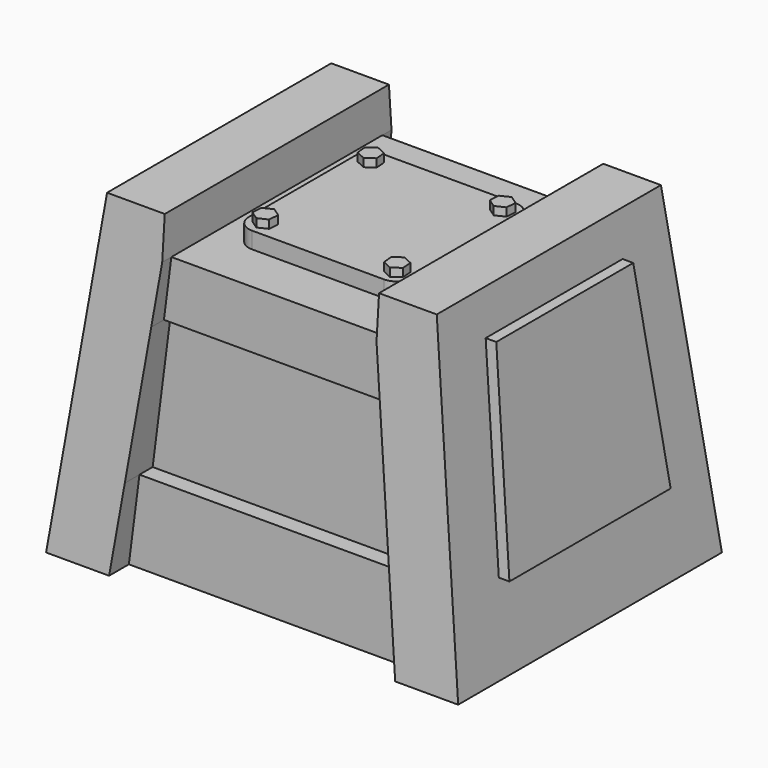
from build123d import *

# Parameters (mm, degrees)
F1_DEPTH  = 40
F2_DEPTH  = 4
F3_DEPTH  = 3
F4_DEPTH  = 5
F6_DEPTH  = 4
F7_DEPTH  = 3
F8_DEPTH  = 5
F10_DEPTH = 2
F13_DEPTH = 50
F15_DEPTH = 1
F16_DEPTH = 50
F17_DEPTH = 40


# Not quite as in the source:
# - ends of sketch curves that miss each other by under 0.0002 mm in the source are joined


with BuildPart() as f1:
    # F0 (on Front) → F1 (new body)
    with BuildSketch(Plane.XZ):
        Polygon((-20, 38.838), (-25, 0), (-17.3563005304, 0), (-16.0689015912, 10), (-13.9011792574, 26.838), (-13, 33.838), (-13, 38.838), align=None)
        Polygon((-16.0689015912, 10), (-17.3563005304, 0), (17.3563005304, 0), (16.0689015912, 10), (0, 10), align=None)
        Polygon((-13.9011792574, 26.838), (-16.0689015912, 10), (0, 10), (16.0689015912, 10), (13.9011792574, 26.838), (-3.37943e-05, 26.838), align=None)
        Polygon((-13, 33.838), (-13.9011792574, 26.838), (3.37943e-05, 26.838), (13.9011792574, 26.838), (13, 33.838), (0, 33.838), align=None)
        Polygon((16.0689015912, 10), (17.3563005304, 0), (25, 0), (20, 38.838), (13, 38.838), (13, 33.838), (13.9011792574, 26.838), align=None)
    extrude(amount=F1_DEPTH)

    # F0 (on Front) → F2 (cut)
    with BuildSketch(Plane.XZ):
        Polygon((-13, 33.838), (-13.9011792574, 26.838), (3.37943e-05, 26.838), (13.9011792574, 26.838), (13, 33.838), (0, 33.838), align=None)
    extrude(amount=F2_DEPTH, mode=Mode.SUBTRACT)

    # F0 (on Front) → F3 (cut)
    with BuildSketch(Plane.XZ):
        Polygon((-16.0689015912, 10), (-17.3563005304, 0), (17.3563005304, 0), (16.0689015912, 10), (0, 10), align=None)
    extrude(amount=F3_DEPTH, mode=Mode.SUBTRACT)

    # F0 (on Front) → F4 (cut)
    with BuildSketch(Plane.XZ):
        Polygon((-13.9011792574, 26.838), (-16.0689015912, 10), (0, 10), (16.0689015912, 10), (13.9011792574, 26.838), (-3.37943e-05, 26.838), align=None)
    extrude(amount=F4_DEPTH, mode=Mode.SUBTRACT)

    # F5 (on face) → F6 (cut)
    with BuildSketch(Plane.XZ.offset(40)):
        Polygon((-13, 33.838), (-13.9011792574, 26.838), (3.37943e-05, 26.838), (13.9011792574, 26.838), (13, 33.838), (0, 33.838), align=None)
    extrude(amount=-F6_DEPTH, mode=Mode.SUBTRACT)

    # F5 (on face) → F7 (cut)
    with BuildSketch(Plane.XZ.offset(40)):
        Polygon((-16.0689015912, 10), (-17.3563005304, 0), (17.3563005304, 0), (16.0689015912, 10), (0, 10), align=None)
    extrude(amount=-F7_DEPTH, mode=Mode.SUBTRACT)

    # F5 (on face) → F8 (cut)
    with BuildSketch(Plane.XZ.offset(40)):
        Polygon((-13.9011792574, 26.838), (-16.0689015912, 10), (0, 10), (16.0689015912, 10), (13.9011792574, 26.838), (-3.37943e-05, 26.838), align=None)
    extrude(amount=-F8_DEPTH, mode=Mode.SUBTRACT)

    # F9 (on face) → F10 (join)
    with BuildSketch(Plane.XY.offset(33.838)):
        with BuildLine():
            ThreePointArc((-10, -28), (-9.4142135624, -29.4142135624), (-8, -30))
            Line((-8, -30), (8, -30))
            ThreePointArc((8, -30), (9.4142135624, -29.4142135624), (10, -28))
            Line((10, -28), (10, -12))
            ThreePointArc((10, -12), (9.4142135624, -10.5857864376), (8, -10))
            Line((8, -10), (-8, -10))
            ThreePointArc((-8, -10), (-9.4142135624, -10.5857864376), (-10, -12))
            Line((-10, -12), (-10, -28))
        make_face()
    extrude(amount=F10_DEPTH)

    # F12 (on face) → F13 (cut)
    with BuildSketch(Plane.YZ.offset(-25)):
        Polygon((-3, 38.838), (0, 0), (0, 38.838), align=None)
        Polygon((-40, 38.838), (-40, 0), (-37, 38.838), align=None)
    extrude(amount=F13_DEPTH, mode=Mode.SUBTRACT)

    # F14 (on face) → F15 (join)
    with BuildSketch(Plane.XY.offset(35.838)):
        Polygon((-7.9011683363, -13.2460867956), (-6.8714413478, -12.5374526663), (-6.9702730115, -11.2913658707), (-8.0988316637, -10.7539132044), (-9.1285586522, -11.4625473337), (-9.0297269885, -12.7086341293), align=None)
        Polygon((6.9702730115, -11.2913658707), (6.8714413478, -12.5374526663), (7.9011683363, -13.2460867956), (9.0297269885, -12.7086341293), (9.1285586522, -11.4625473337), (8.0988316637, -10.7539132044), align=None)
        Polygon((7.9011683363, -26.7539132044), (6.8714413478, -27.4625473337), (6.9702730115, -28.7086341293), (8.0988316637, -29.2460867956), (9.1285586522, -28.5374526663), (9.0297269885, -27.2913658707), align=None)
        Polygon((-6.9702730115, -28.7086341293), (-6.8714413478, -27.4625473337), (-7.9011683363, -26.7539132044), (-9.0297269885, -27.2913658707), (-9.1285586522, -28.5374526663), (-8.0988316637, -29.2460867956), align=None)
    extrude(amount=F15_DEPTH)

    # F12 (on face) → F16 (join)
    with BuildSketch(Plane.YZ.offset(-25)):
        Polygon((-20, 33.838), (-30.3862196818, 33.838), (-32.2275606365, 10), (-20, 10), (-7.7724393635, 10), (-9.6137803182, 33.838), align=None)
    extrude(amount=F16_DEPTH)

    # F0 (on Front) → F17 (cut)
    with BuildSketch(Plane.XZ):
        Polygon((-25, 38.838), (-25, 10), (-21.2873989392, 38.838), align=None)
        Polygon((21.2873989392, 38.838), (25, 10), (25, 38.838), align=None)
    extrude(amount=F17_DEPTH, mode=Mode.SUBTRACT)


solid = f1.part
